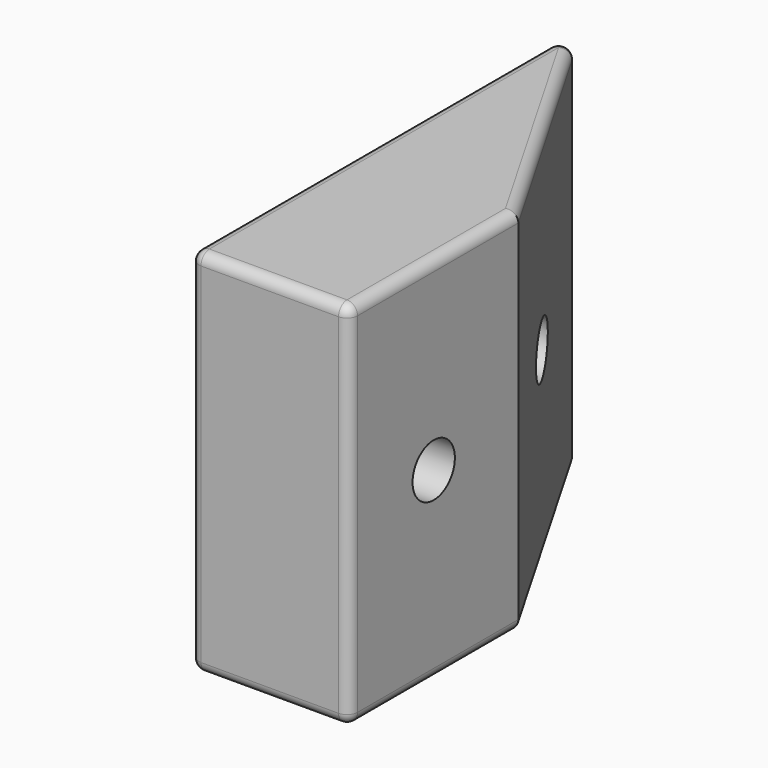
from build123d import *

# Parameters (mm, degrees)
F1_DEPTH       = 44.45
F3_D           = 6.35
F3_CSINK_D     = 10.16
F3_CSINK_ANGLE = 82
F4_T1_DEPTH    = 68.1485226281
F5_R           = 1.27


# Not quite as in the source:
# - a fillet or chamfer that OpenCascade refuses, or shapes differently, is made with other operations: its cross-section is extruded or revolved along the edge and cut away or added
# - a feature names something its author has since deleted; it is built from what else it names


with BuildPart() as f1:
    # F0 (on Top) → F1 (new body)
    with BuildSketch(Plane.XY):
        Polygon((0, 58.3955678842), (0, 0), (19.05, 0), (19.05, 25.4), align=None)
    extrude(amount=F1_DEPTH)

    # F3 (through all)
    with Locations(Plane(origin=(0, 0, 0), x_dir=(0, -1, 0), z_dir=(-1, 0, 0))):
        with Locations((-12.7, 22.225), (-38.1, 22.225)):
            CounterSinkHole(F3_D / 2, F3_CSINK_D / 2, counter_sink_angle=F3_CSINK_ANGLE)

    # F4: fillet of radius 1.27 on 1 edges, made by hand

    # F4_s2 → F4_t1 (cut)
    with BuildSketch(Plane.XY.offset(-11.849261314)):
        with BuildLine():
            ThreePointArc((0, 53.6558633586), (0.9412998127, 54.882589158), (2.3698522628, 54.2908633586))
            Line((2.3698522628, 54.2908633586), (0, 58.3955678842))
            Line((0, 58.3955678842), (0, 53.6558633586))
        make_face()
    extrude(amount=F4_T1_DEPTH, mode=Mode.SUBTRACT)

    # F5
    f5_edges = [f1.edges().sort_by_distance(p)[0] for p in [
        (0.9413, 54.882589, 44.45),
        (10.709926, 39.845432, 44.45),
        (19.05, 12.7, 44.45),
        (9.525, 0, 44.45),
        (0, 26.827932, 44.45),
        (0.9413, 54.882589, 0),
        (10.709926, 39.845432, 0),
        (19.05, 12.7, 0),
        (9.525, 0, 0),
        (0, 26.827932, 0),
        (0, 0, 22.225),
        (19.05, 0, 22.225),
    ]]
    fillet(f5_edges, radius=F5_R)


solid = f1.part
